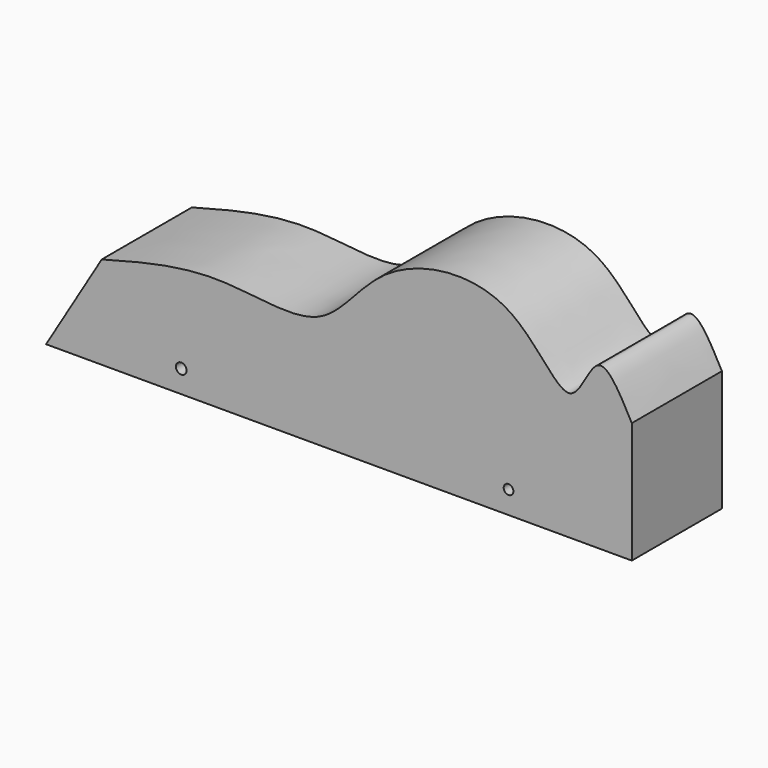
from build123d import *

# Parameters (mm, degrees)
F0_R     = 1.180077203
F0_R_2   = 1.075
F1_DEPTH = 25
F2_DEPTH = 25
F3_DEPTH = 156


# Not quite as in the source:
# - an extrude ends at something that could not be found from the text; its depth is read off the source's solid


with BuildPart() as f1:
    # F0 (on Front) → F1 (new body)
    with BuildSketch(Plane.XZ):
        with BuildLine():
            Line((-80, -25), (-50, -25))
            Line((-50, -25), (22.6452976465, -25))
            Line((22.6452976465, -25), (50, -25))
            Line((50, -25), (50, 1.8597864546))
            add(Edge.make_bspline(
                [(-67.6445906489, -4.4076510815), (-59.0102886259, -2.1011168124), (-42.5071210423, 2.3074759699), (-17.5616744307, -4.6627715865), (-6.6736378345, 16.9872606787), (24.059206598, 21.3213776549), (36.3958726575, -3.9761585615), (42.342577975, 16.1775178738), (47.3665093795, 6.7838472254), (50, 1.8597864546)],
                knots=[0, 0, 0, 0, 0.1696918572, 0.3243404215, 0.4741260658, 0.6448671709, 0.7855029125, 0.8875629417, 1, 1, 1, 1], degree=3))
            Line((-67.6445906489, -4.4076510815), (-80, -25))
        make_face()
        with Locations((-50, -20)):
            Circle(F0_R, mode=Mode.SUBTRACT)
        with Locations((22.6452976465, -20)):
            Circle(F0_R_2, mode=Mode.SUBTRACT)
    extrude(amount=F1_DEPTH)

    # F0 (on Front) → F2 (join)
    with BuildSketch(Plane.XZ):
        with BuildLine():
            Line((-80, -25), (-50, -25))
            Line((-50, -25), (22.6452976465, -25))
            Line((22.6452976465, -25), (50, -25))
            Line((50, -25), (50, 1.8597864546))
            add(Edge.make_bspline(
                [(-67.6445906489, -4.4076510815), (-59.0102886259, -2.1011168124), (-42.5071210423, 2.3074759699), (-17.5616744307, -4.6627715865), (-6.6736378345, 16.9872606787), (24.059206598, 21.3213776549), (36.3958726575, -3.9761585615), (42.342577975, 16.1775178738), (47.3665093795, 6.7838472254), (50, 1.8597864546)],
                knots=[0, 0, 0, 0, 0.1696918572, 0.3243404215, 0.4741260658, 0.6448671709, 0.7855029125, 0.8875629417, 1, 1, 1, 1], degree=3))
            Line((-67.6445906489, -4.4076510815), (-80, -25))
        make_face()
        with Locations((-50, -20)):
            Circle(F0_R, mode=Mode.SUBTRACT)
        with Locations((22.6452976465, -20)):
            Circle(F0_R_2, mode=Mode.SUBTRACT)
    extrude(amount=F2_DEPTH)

    # F0 (on Front) → F3 (cut, through all)
    with BuildSketch(Plane.XZ):
        with BuildLine():
            Line((-50, 25), (-67.6445906489, -4.4076510815))
            add(Edge.make_bspline(
                [(-67.6445906489, -4.4076510815), (-59.0102886259, -2.1011168124), (-42.5071210423, 2.3074759699), (-17.5616744307, -4.6627715865), (-6.6736378345, 16.9872606787), (24.059206598, 21.3213776549), (36.3958726575, -3.9761585615), (42.342577975, 16.1775178738), (47.3665093795, 6.7838472254), (50, 1.8597864546)],
                knots=[0, 0, 0, 0, 0.1696918572, 0.3243404215, 0.4741260658, 0.6448671709, 0.7855029125, 0.8875629417, 1, 1, 1, 1], degree=3))
            Line((50, 1.8597864546), (50, 25))
            Line((50, 25), (-50, 25))
        make_face()
    extrude(amount=-F3_DEPTH, mode=Mode.SUBTRACT)


solid = f1.part
